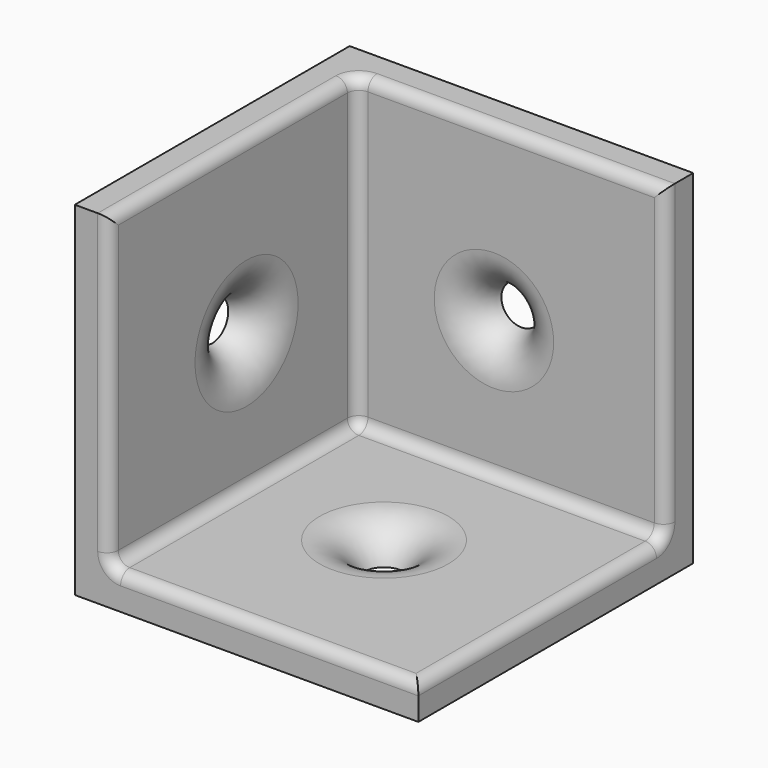
from build123d import *

# Parameters (mm, degrees)
F1_W     = 30
F1_H     = 30
F1_R     = 1.75
F2_DEPTH = 3
F0_W     = 30
F0_H     = 30
F0_R     = 1.75
F3_DEPTH = 3
F5_W     = 30
F5_H     = 30
F5_R     = 1.75
F6_DEPTH = 3
F7_R     = 1


# Not quite as in the source:
# - a fillet or chamfer that OpenCascade refuses, or shapes differently, is made with other operations: its cross-section is extruded or revolved along the edge and cut away or added


with BuildPart() as f2:
    # F1 (on Right) → F2 (new body)
    with BuildSketch(Plane.YZ):
        with Locations((15, 15)):
            Rectangle(F1_W, F1_H)
        with Locations((15, 15)):
            Circle(F1_R, mode=Mode.SUBTRACT)
    extrude(amount=F2_DEPTH)

    # F0 (on Top) → F3 (join)
    with BuildSketch(Plane.XY):
        with Locations((15, 15)):
            Rectangle(F0_W, F0_H)
        with Locations((15, 15)):
            Circle(F0_R, mode=Mode.SUBTRACT)
    extrude(amount=F3_DEPTH)

    # F5 (on face) → F6 (join)
    with BuildSketch(Plane.XZ.offset(-30)):
        with Locations((15, 15)):
            Rectangle(F5_W, F5_H)
        with Locations((15, 15)):
            Circle(F5_R, mode=Mode.SUBTRACT)
    extrude(amount=F6_DEPTH)

    # F7
    f7_edges = [f2.edges().sort_by_distance(p)[0] for p in [
        (3, 13.5, 3),
        (3, 13.5, 30),
        (30, 13.5, 3),
        (3, 0, 16.5),
        (16.5, 0, 3),
        (16.5, 27, 3),
        (16.5, 27, 30),
        (3, 27, 16.5),
        (30, 27, 16.5),
    ]]
    fillet(f7_edges, radius=F7_R)

    # F8: fillet of radius 4 on 1 edges, made by hand

    # F8_s1 → F8_t2 (revolve, cut)
    with BuildSketch(Plane.XZ.offset(-15)):
        with BuildLine():
            ThreePointArc((16.75, 0), (18.1734936034, 2.1622776602), (20.6229833462, 3))
            Line((20.6229833462, 3), (16.75, 3))
            Line((16.75, 3), (16.75, 0))
        make_face()
    revolve(axis=Axis((15, 15, 3), (0, 0, 1)), mode=Mode.SUBTRACT)

    # F9: fillet of radius 4 on 1 edges, made by hand

    # F9_s1 → F9_t2 (revolve, cut)
    with BuildSketch(Plane.XY.offset(15)):
        with BuildLine():
            ThreePointArc((3, 20.6229833462), (2.1622776602, 18.1734936034), (0, 16.75))
            Line((0, 16.75), (3, 16.75))
            Line((3, 16.75), (3, 20.6229833462))
        make_face()
    revolve(axis=Axis((3, 15, 15), (1, 0, 0)), mode=Mode.SUBTRACT)

    # F10: fillet of radius 3.5 on 1 edges, made by hand

    # F10_s1 → F10_t2 (revolve, cut)
    with BuildSketch(Plane.XY.offset(15)):
        with BuildLine():
            ThreePointArc((20.2141016151, 27), (17.9228137677, 27.8542486889), (16.75, 30))
            Line((16.75, 30), (16.75, 27))
            Line((16.75, 27), (20.2141016151, 27))
        make_face()
    revolve(axis=Axis((15, 27, 15), (0, -1, 0)), mode=Mode.SUBTRACT)


solid = f2.part
